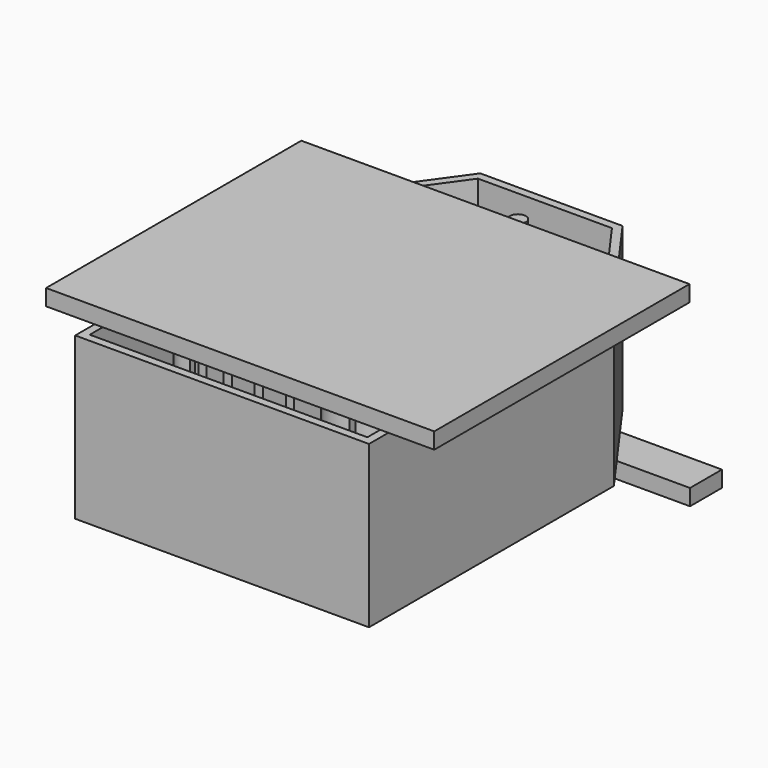
from build123d import *

# Parameters (mm, degrees)
F1_DEPTH     = 25.4
F2_R         = 1.27
F3_DEPTH     = 25.4
F4_W         = 61.0795281827
F4_H         = 6.2752962112
F5_DEPTH     = 2.54
F6_TEXT_SIZE = 17.5724968988
F7_TEXT_SIZE = 15.6665771388
F8_DEPTH     = 25.4
F9_W         = 61.0795281827
F9_H         = 50.2023547888
F10_DEPTH    = 2.54


# Not quite as in the source:
# - Text() gives the source's letters only with a copy of the font that has no kerning and outlines rounded to 1/6400 em; it was checked with that copy


with BuildPart() as f1:
    # F0 (on Top) → F1 (new body)
    with BuildSketch(Plane.XY):
        Polygon((-11.1927306941, 45.687792372), (-23.114, 29.0783834514), (-23.114, -19.082207628), (23.114, -19.082207628), (23.114, 29.0783834514), (11.1927306941, 45.687792372), align=None)
        Polygon((-10.541, 44.417792372), (0, 44.417792372), (10.541, 44.417792372), (21.844, 28.669792372), (21.844, -17.812207628), (0, -17.812207628), (-21.844, -17.812207628), (-21.844, 28.669792372), align=None, mode=Mode.SUBTRACT)
    extrude(amount=F1_DEPTH)


with BuildPart() as f3:
    # F2 (on Top) → F3 (new body)
    with BuildSketch(Plane.XY):
        with Locations((0, 39.083792372)):
            Circle(F2_R)
    extrude(amount=F3_DEPTH)


with BuildPart() as f5:
    # F4 (on face) → F5 (new body)
    with BuildSketch(Plane(origin=(0, 0, 0), x_dir=(1, 0, 0), z_dir=(0, 0, -1))):
        with Locations((0.2091769129, -37.6517660916)):
            Rectangle(F4_W, F4_H)
    extrude(amount=F5_DEPTH)


with BuildPart() as f8:
    # F6 (on Top) + F7 (on Top) → F8 (new body)
    with BuildSketch(Plane.XY):
        with Locations((-15.494, 2.6684892792)):
            Text('Tea', F6_TEXT_SIZE, font='Open Sans', font_style=FontStyle.BOLD, text_align=(TextAlign.LEFT, TextAlign.BOTTOM))
    with BuildSketch(Plane.XY):
        with Locations((-15.494, -11.2799355399)):
            Text('time', F7_TEXT_SIZE, font='Open Sans', font_style=FontStyle.ITALIC, text_align=(TextAlign.LEFT, TextAlign.BOTTOM))
    extrude(amount=F8_DEPTH)


with BuildPart() as f10:
    # F9 (on face) → F10 (new body)
    with BuildSketch(Plane.XY.offset(25.4)):
        with Locations((-0.2091769129, 9.8312944174)):
            Rectangle(F9_W, F9_H)
    extrude(amount=F10_DEPTH)


solid = Compound([f1.part, f3.part, f5.part, f8.part, f10.part])
